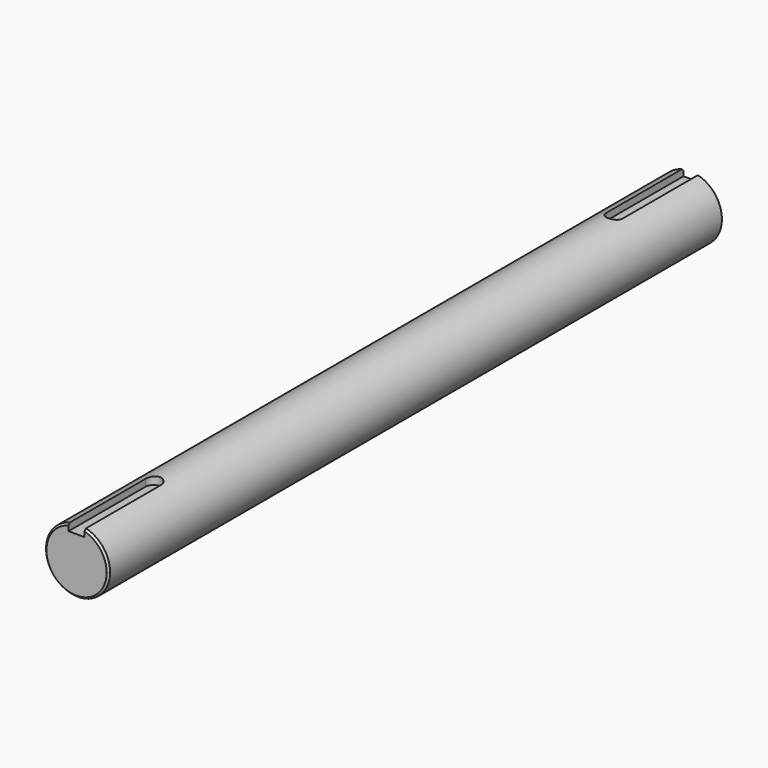
from build123d import *

# Parameters (mm, degrees)
F0_R     = 12.7
F1_DEPTH = 152.4
F4_DEPTH = 3.175
F5_SIZE  = 0.762
F6_SIZE  = 0.762


# Not quite as in the source:
# - a pattern or mirror of a feature is missing from the dataset's text; its kind, count and spacing are read off the source's solid


with BuildPart() as f1:
    # F0 (on Front) → F1 (new body, symmetric)
    with BuildSketch(Plane.XZ):
        Circle(F0_R)
    extrude(amount=F1_DEPTH, both=True)

    # F3 (on offset) → F4 (cut)
    with BuildSketch(Plane.XY.offset(12.7)):
        with BuildLine():
            Line((3.175, -156.7815), (3.175, -114.3))
            ThreePointArc((3.175, -114.3), (0, -111.125), (-3.175, -114.3))
            Line((-3.175, -114.3), (-3.175, -156.7815))
            Line((-3.175, -156.7815), (3.175, -156.7815))
        make_face()
    f4 = extrude(amount=-F4_DEPTH, mode=Mode.SUBTRACT)

    # F4_copies: F4 across plane
    add(f4.mirror(Plane.ZX), mode=Mode.SUBTRACT)

    # F5
    f5_edges = [f1.edges().sort_by_distance(p)[0] for p in [
        (-7.77713, -152.4, -10.040232),
    ]]
    chamfer(f5_edges, length=F5_SIZE)

    # F6
    f6_edges = [f1.edges().sort_by_distance(p)[0] for p in [
        (-7.77713, 152.4, -10.040232),
        (10.040232, 152.4, 7.77713),
    ]]
    chamfer(f6_edges, length=F6_SIZE)


solid = f1.part
